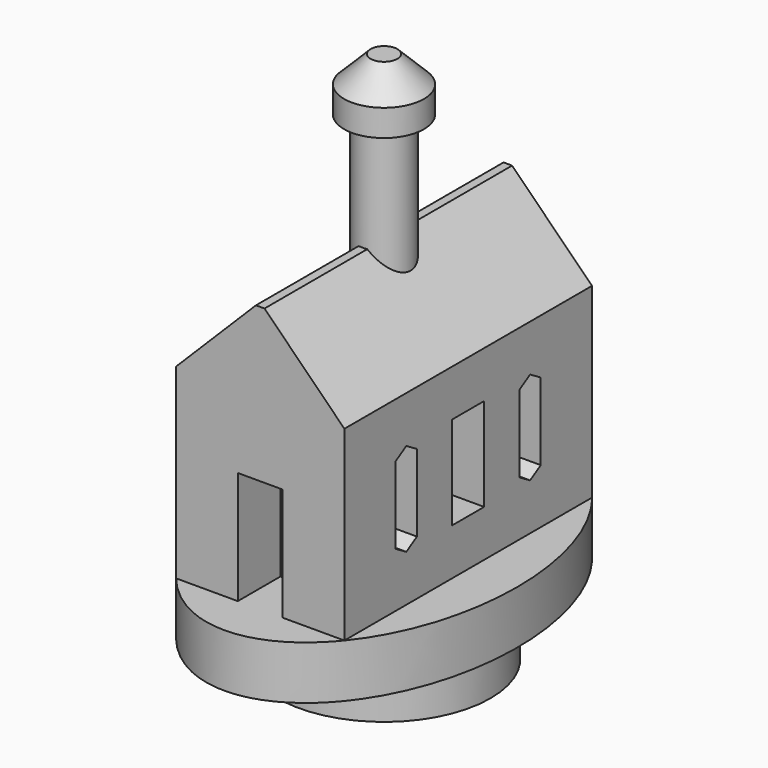
from build123d import *

# Parameters (mm, degrees)
F0_R          = 10.16
F1_DEPTH      = 5.08
F3_DEPTH      = 5.08
F4_W          = 16.0591960874
F4_H          = 29.5184687494
F5_DEPTH      = 25.4
F6_R          = 2.54
F7_DEPTH      = 10.16
F8_R          = 3.81
F9_DEPTH      = 5.08
F10_SIZE      = 2.54
F11_T4_DEPTH  = 68.710917486
F11_S5_R      = 2.54
F11_T6_DEPTH  = 36
F11_T10_DEPTH = 68.710917486
F11_S11_R     = 2.54
F11_T12_DEPTH = 36
F12_W         = 4.2759752832
F12_H         = 10.7621589082
F13_DEPTH     = 5.08
F15_DEPTH     = 5.08
F17_DEPTH     = 5.08
F19_DEPTH     = 5.08


# Not quite as in the source:
# - a fillet or chamfer that OpenCascade refuses, or shapes differently, is made with other operations: its cross-section is extruded or revolved along the edge and cut away or added


with BuildPart() as f1:
    # F0 (on Top) → F1 (new body)
    with BuildSketch(Plane.XY):
        Circle(F0_R)
    extrude(amount=F1_DEPTH)

    # F2 (on face) → F3 (join)
    with BuildSketch(Plane.XY.offset(5.08)):
        with BuildLine():
            add(Edge.make_bspline(
                [(0, 19.05), (-21.9970452561, 19.05), (-10.9985226281, -9.525), (0, -38.1), (10.9985226281, -9.525), (21.9970452561, 19.05), (0, 19.05)],
                knots=[0, 0, 0, 2.0943951024, 2.0943951024, 4.1887902048, 4.1887902048, 6.2831853072, 6.2831853072, 6.2831853072], degree=2, weights=[1, 0.5, 1, 0.5, 1, 0.5, 1]))
        make_face()
    extrude(amount=F3_DEPTH)

    # F4 (on face) → F5 (join)
    with BuildSketch(Plane.XY.offset(10.16)):
        Rectangle(F4_W, F4_H)
    extrude(amount=F5_DEPTH)

    # F6 (on face) → F7 (join)
    with BuildSketch(Plane.XY.offset(35.56)):
        Circle(F6_R)
    extrude(amount=F7_DEPTH)

    # F8 (on face) → F9 (join)
    with BuildSketch(Plane.XY.offset(45.72)):
        Circle(F8_R)
    extrude(amount=F9_DEPTH)

    # F10
    f10_edges = [f1.edges().sort_by_distance(p)[0] for p in [
        (-3.81, 0, 50.8),
    ]]
    chamfer(f10_edges, length=F10_SIZE)

    # F11: chamfer of 7.62 on 2 edges, made by hand


with BuildPart() as f11_tool2:
    # F11_s3 → F11_t4 (new body)
    with BuildSketch(Plane.XZ.offset(34.355458743)):
        with BuildLine():
            Line((0.1940718968, 35.7755261469), (8.2451241906, 27.7244738531))
            Line((8.2451241906, 27.7244738531), (8.3975241906, 27.7244738531))
            ThreePointArc((8.3975241906, 27.7244738531), (8.1819980437, 31.6422369265), (8.1819980437, 35.56))
            Line((8.1819980437, 35.56), (8.0295980437, 35.7124))
            ThreePointArc((8.0295980437, 35.7124), (4.1118349703, 35.7124), (0.1940718968, 35.9279261469))
            Line((0.1940718968, 35.9279261469), (0.1940718968, 35.7755261469))
        make_face()
    extrude(amount=-F11_T4_DEPTH)

    # F11_s5 → F11_t6 (cut, symmetric)
    with BuildSketch(Plane.XY.offset(31.8)):
        Circle(F11_S5_R)
    extrude(amount=F11_T6_DEPTH, both=True, mode=Mode.SUBTRACT)


with BuildPart() as f1_1:
    add(f1.part)

    # F11_t1: cut F11_tool2
    add(f11_tool2.part, mode=Mode.SUBTRACT)


with BuildPart() as f11_tool8:
    # F11_s9 → F11_t10 (new body)
    with BuildSketch(Plane.XZ.offset(-34.355458743)):
        with BuildLine():
            Line((-0.1940718968, 35.7755261469), (-8.2451241906, 27.7244738531))
            Line((-8.2451241906, 27.7244738531), (-8.3975241906, 27.7244738531))
            ThreePointArc((-8.3975241906, 27.7244738531), (-8.1819980437, 31.6422369265), (-8.1819980437, 35.56))
            Line((-8.1819980437, 35.56), (-8.0295980437, 35.7124))
            ThreePointArc((-8.0295980437, 35.7124), (-4.1118349703, 35.7124), (-0.1940718968, 35.9279261469))
            Line((-0.1940718968, 35.9279261469), (-0.1940718968, 35.7755261469))
        make_face()
    extrude(amount=F11_T10_DEPTH)

    # F11_s11 → F11_t12 (cut, symmetric)
    with BuildSketch(Plane.XY.offset(31.8)):
        Circle(F11_S11_R)
    extrude(amount=F11_T12_DEPTH, both=True, mode=Mode.SUBTRACT)


with BuildPart() as f1_2:
    add(f1_1.part)

    # F11_t7: cut F11_tool8
    add(f11_tool8.part, mode=Mode.SUBTRACT)

    # F12 (on face) → F13 (cut)
    with BuildSketch(Plane.XZ.offset(14.7592343747)):
        with Locations((0, 15.5410794541)):
            Rectangle(F12_W, F12_H)
    extrude(amount=-F13_DEPTH, mode=Mode.SUBTRACT)

    # F14 (on face) → F15 (cut)
    with BuildSketch(Plane(origin=(0, 14.7592343747, 0), x_dir=(-1, 0, 0), z_dir=(0, 1, 0))):
        with BuildLine():
            ThreePointArc((1.483647583, 29.810695909), (0, 29.332343272), (-1.483647583, 29.810695909))
            ThreePointArc((-1.483647583, 29.810695909), (-1.1582605793, 25.4885104617), (2.54, 27.749048546))
            ThreePointArc((2.54, 27.749048546), (2.2605380843, 28.9073091253), (1.483647583, 29.810695909))
        make_face()
        with BuildLine():
            ThreePointArc((1.483647583, 29.810695909), (0, 30.289048546), (-1.483647583, 29.810695909))
            ThreePointArc((-1.483647583, 29.810695909), (0, 29.332343272), (1.483647583, 29.810695909))
        make_face()
    extrude(amount=-F15_DEPTH, mode=Mode.SUBTRACT)

    # F16 (on face) → F17 (cut)
    with BuildSketch(Plane.YZ.offset(8.0295980437)):
        Polygon((-7.3796171873, 19.05), (-7.3796171873, 23.495), (-8.6496171873, 22.7300348458), (-8.6496171873, 19.05), align=None)
        Polygon((-6.1096171873, 22.7300348458), (-7.3796171873, 23.495), (-7.3796171873, 19.05), (-6.1096171873, 19.05), align=None)
        Polygon((-6.1096171873, 19.05), (-7.3796171873, 19.05), (-7.3796171873, 14.605), (-6.1096171873, 15.3699651542), align=None)
        Polygon((-7.3796171873, 14.605), (-7.3796171873, 19.05), (-8.6496171873, 19.05), (-8.6496171873, 15.3699651542), align=None)
        Polygon((0, 19.05), (0, 23.495), (-1.905, 23.495), (-1.905, 20.1974477314), align=None)
        Polygon((1.905, 23.495), (0, 23.495), (0, 19.05), (1.905, 20.1974477314), align=None)
        Polygon((-1.905, 19.05), (0, 19.05), (-1.905, 20.1974477314), align=None)
        Polygon((1.905, 20.1974477314), (0, 19.05), (1.905, 19.05), align=None)
        Polygon((1.905, 19.05), (0, 19.05), (1.905, 17.9025522686), align=None)
        Polygon((1.905, 17.9025522686), (0, 19.05), (0, 14.605), (1.905, 14.605), align=None)
        Polygon((0, 14.605), (0, 19.05), (-1.905, 17.9025522686), (-1.905, 14.605), align=None)
        Polygon((-1.905, 17.9025522686), (0, 19.05), (-1.905, 19.05), align=None)
        Polygon((7.3796171873, 14.605), (7.3796171873, 19.05), (6.1096171873, 19.05), (6.1096171873, 15.3699651542), align=None)
        Polygon((7.3796171873, 14.605), (8.6496171873, 15.3699651542), (8.6496171873, 19.05), (7.3796171873, 19.05), align=None)
        Polygon((8.6496171873, 22.7300348458), (7.3796171873, 23.495), (7.3796171873, 19.05), (8.6496171873, 19.05), align=None)
        Polygon((7.3796171873, 19.05), (7.3796171873, 23.495), (6.1096171873, 22.7300348458), (6.1096171873, 19.05), align=None)
    extrude(amount=-F17_DEPTH, mode=Mode.SUBTRACT)

    # F18 (on face) → F19 (cut)
    with BuildSketch(Plane(origin=(-8.0295980437, 0, 0), x_dir=(0, -1, 0), z_dir=(-1, 0, 0))):
        Polygon((-6.1096171873, 19.05), (-7.3796171873, 19.05), (-7.3796171873, 14.605), (-6.1096171873, 15.3699651542), align=None)
        Polygon((-7.3796171873, 19.05), (-7.3796171873, 23.495), (-8.6496171873, 22.7300348458), (-8.6496171873, 19.05), align=None)
        Polygon((0, 19.05), (0, 23.622), (-1.905, 23.622), (-1.905, 20.1974477314), align=None)
        Polygon((-1.905, 19.05), (0, 19.05), (-1.905, 20.1974477314), align=None)
        Polygon((-1.905, 17.9025522686), (0, 19.05), (-1.905, 19.05), align=None)
        Polygon((0, 14.478), (0, 19.05), (-1.905, 17.9025522686), (-1.905, 14.478), align=None)
        Polygon((1.905, 17.9025522686), (0, 19.05), (0, 14.478), (1.905, 14.478), align=None)
        Polygon((1.905, 19.05), (0, 19.05), (1.905, 17.9025522686), align=None)
        Polygon((1.905, 20.1974477314), (0, 19.05), (1.905, 19.05), align=None)
        Polygon((1.905, 23.622), (0, 23.622), (0, 19.05), (1.905, 20.1974477314), align=None)
        Polygon((7.3796171873, 19.05), (7.3796171873, 23.495), (6.1096171873, 22.7300348458), (6.1096171873, 19.05), align=None)
        Polygon((8.6496171873, 22.7300348458), (7.3796171873, 23.495), (7.3796171873, 19.05), (8.6496171873, 19.05), align=None)
        Polygon((7.3796171873, 14.605), (7.3796171873, 19.05), (6.1096171873, 19.05), (6.1096171873, 15.3699651542), align=None)
        Polygon((-6.1096171873, 22.7300348458), (-7.3796171873, 23.495), (-7.3796171873, 19.05), (-6.1096171873, 19.05), align=None)
        Polygon((-8.6496171873, 19.05), (-8.6496171873, 15.3699651542), (-7.3796171873, 14.605), (-7.3796171873, 19.05), align=None)
        Polygon((8.6496171873, 19.05), (7.3796171873, 19.05), (7.3796171873, 14.605), (8.6496171873, 15.3699651542), align=None)
    extrude(amount=-F19_DEPTH, mode=Mode.SUBTRACT)


solid = f1_2.part
